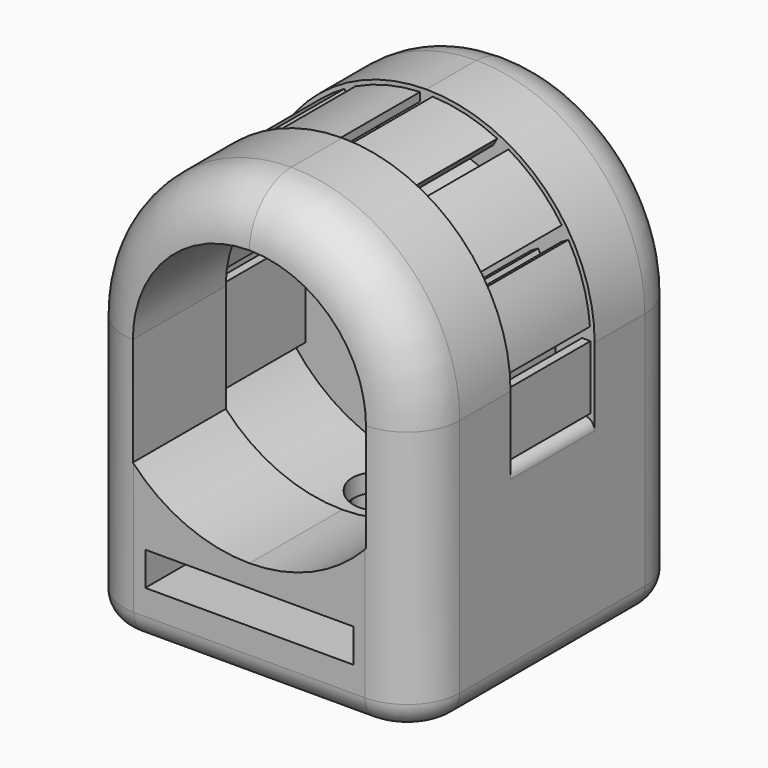
from build123d import *

# Parameters (mm, degrees)
F0_W          = 20.32
F0_H          = 20.32
F1_DEPTH      = 26.162
F2_R          = 10.15999
F3_R          = 3.2512
F4_DEPTH      = 20.321
F7_DEPTH      = 13.3604
F9_DEPTH      = 6.35
F10_R         = 0.635
F11_R         = 3.2512
F12_DEPTH     = 4.826
F13_R         = 1.905
F14_DEPTH     = 25.4
F16_W         = 12.573
F16_H         = 2.032
F17_DEPTH     = 16.51
F18_R         = 1.0795
F19_DEPTH     = 5.08
F20_T1_DEPTH  = 23.93951
F20_T3_DEPTH  = 2e-05
F20_T6_ANGLE  = 90
F20_T8_ANGLE  = 90
F20_T10_ANGLE = 90
F20_T12_ANGLE = 90
F21_R         = 1.524
F22_W         = 0.508
F22_H         = 3.8441118483
F22_H_2       = 5.6562280912
F23_DEPTH     = 6.35
F25_DEPTH     = 4.826


# Not quite as in the source:
# - a fillet or chamfer that OpenCascade refuses, or shapes differently, is made with other operations: its cross-section is extruded or revolved along the edge and cut away or added
# - a fillet or chamfer is up to 0.001 mm smaller than in the source, because OpenCascade refuses the exact size


with BuildPart() as f1:
    # F0 (on Top) → F1 (new body)
    with BuildSketch(Plane.XY):
        Rectangle(F0_W, F0_H)
    extrude(amount=F1_DEPTH)

    # F2 (radius 10.16 in the source; OpenCascade refuses exactly that, so slightly less here)
    f2_edges = [f1.edges().sort_by_distance(p)[0] for p in [
        (10.16, 0, 26.162),
        (-10.16, 0, 26.162),
    ]]
    fillet(f2_edges, radius=F2_R)

    # F3 (on face) → F4 (cut, through all)
    with BuildSketch(Plane.XZ.offset(10.16)):
        with Locations((0, 16.002)):
            Circle(F3_R)
    extrude(amount=-F4_DEPTH, mode=Mode.SUBTRACT)

    # F6 (on face) → F7 (cut)
    with BuildSketch(Plane.XZ.offset(10.16)):
        with BuildLine():
            ThreePointArc((7.0358, 16.002), (0, 23.0378), (-7.0358, 16.002))
            Line((-7.0358, 16.002), (-7.0358, 9.4689639676))
            ThreePointArc((-7.0358, 9.4689639676), (-3.8378415735, 7.2012038146), (0, 6.4008))
            ThreePointArc((0, 6.4008), (3.8378415735, 7.2012038146), (7.0358, 9.4689639676))
            Line((7.0358, 9.4689639676), (7.0358, 16.002))
        make_face()
    extrude(amount=-F7_DEPTH, mode=Mode.SUBTRACT)

    # F8 (on face) → F9 (cut)
    with BuildSketch(Plane.XZ.offset(-3.2004)):
        with BuildLine():
            Line((-12.8970071673, 11.938), (-9.1174678963, 11.938))
            ThreePointArc((-9.1174678963, 11.938), (0, 6.0198), (9.1174678963, 11.938))
            Line((9.1174678963, 11.938), (12.2319469228, 11.938))
            Line((12.2319469228, 11.938), (12.2319469228, 29.744040221))
            Line((12.2319469228, 29.744040221), (-12.8970071673, 29.744040221))
            Line((-12.8970071673, 29.744040221), (-12.8970071673, 11.938))
        make_face()
        with BuildLine():
            Line((7.0358, 16.002), (7.0358, 9.4689639676))
            ThreePointArc((7.0358, 9.4689639676), (0, 6.4008), (-7.0358, 9.4689639676))
            Line((-7.0358, 9.4689639676), (-7.0358, 16.002))
            ThreePointArc((-7.0358, 16.002), (0, 23.0378), (7.0358, 16.002))
        make_face(mode=Mode.SUBTRACT)
    extrude(amount=F9_DEPTH, mode=Mode.SUBTRACT)

    # F10
    f10_edges = [f1.edges().sort_by_distance(p)[0] for p in [
        (9.117468, 0.0254, 11.938),
        (10.16, 0.0254, 11.938),
        (-9.117468, 0.0254, 11.938),
        (-10.16, 0.0254, 11.938),
    ]]
    fillet(f10_edges, radius=F10_R)

    # F11 (on face) → F12 (cut)
    with BuildSketch(Plane(origin=(0, 10.16, 0), x_dir=(-1, 0, 0), z_dir=(0, 1, 0))):
        Polygon((-0.0026727509, 9.8428279082), (5.3326631223, 12.920099284), (5.3353358732, 19.0792713758), (0.0026727509, 22.1611720918), (-5.3326631223, 19.083900716), (-5.3353358732, 12.9247286242), align=None)
        with Locations((0, 16.002)):
            Circle(F11_R, mode=Mode.SUBTRACT)
    extrude(amount=-F12_DEPTH, mode=Mode.SUBTRACT)

    # F13 (on face) → F14 (cut)
    with BuildSketch(Plane(origin=(0, 0, 0), x_dir=(1, 0, 0), z_dir=(0, 0, -1))):
        Circle(F13_R)
    extrude(amount=-F14_DEPTH, mode=Mode.SUBTRACT)

    # F16 (on face) → F17 (cut)
    with BuildSketch(Plane.XZ.offset(10.16)):
        with Locations((0, 4.064)):
            Rectangle(F16_W, F16_H)
    extrude(amount=-F17_DEPTH, mode=Mode.SUBTRACT)

    # F18 (on face) → F19 (cut, through all)
    with BuildSketch(Plane(origin=(0, 0, 0), x_dir=(1, 0, 0), z_dir=(0, 0, -1))):
        with Locations((3.2688132281, 3.2688132281)):
            Circle(F18_R)
        with Locations((-3.2688132281, 3.2688132281)):
            Circle(F18_R)
        with Locations((-3.2688132281, -3.2688132281)):
            Circle(F18_R)
        with Locations((3.2688132281, -3.2688132281)):
            Circle(F18_R)
    extrude(amount=-F19_DEPTH, mode=Mode.SUBTRACT)

    # F20: fillet of radius 3.175 on 2 edges, made by hand

    # F20_s2 → F20_t1 (cut)
    with BuildSketch(Plane.XY.offset(-7.9375)):
        with BuildLine():
            ThreePointArc((-10.16, 6.985), (-9.2300640303, 9.2300640303), (-6.985, 10.16))
            Line((-6.985, 10.16), (-10.16, 10.16))
            Line((-10.16, 10.16), (-10.16, 6.985))
        make_face()
        with BuildLine():
            ThreePointArc((6.985, 10.16), (9.2300640303, 9.2300640303), (10.16, 6.985))
            Line((10.16, 6.985), (10.16, 10.16))
            Line((10.16, 10.16), (6.985, 10.16))
        make_face()
        with BuildLine():
            ThreePointArc((6.985, -10.16), (9.2300640303, -9.2300640303), (10.16, -6.985))
            Line((10.16, -6.985), (10.16, -10.16))
            Line((10.16, -10.16), (6.985, -10.16))
        make_face()
        with BuildLine():
            ThreePointArc((-10.16, -6.985), (-9.2300640303, -9.2300640303), (-6.985, -10.16))
            Line((-6.985, -10.16), (-10.16, -10.16))
            Line((-10.16, -10.16), (-10.16, -6.985))
        make_face()
    extrude(amount=F20_T1_DEPTH, mode=Mode.SUBTRACT)

    # F20_s4 → F20_t3 (cut)
    with BuildSketch(Plane.YZ.offset(-1e-05)):
        with BuildLine():
            ThreePointArc((10.16, 22.987), (9.2300640303, 25.2320640303), (6.985, 26.162))
            Line((6.985, 26.162), (10.16, 26.162))
            Line((10.16, 26.162), (10.16, 22.987))
        make_face()
        with BuildLine():
            ThreePointArc((-10.16, 22.987), (-9.2300640303, 25.2320640303), (-6.985, 26.162))
            Line((-6.985, 26.162), (-10.16, 26.162))
            Line((-10.16, 26.162), (-10.16, 22.987))
        make_face()
    extrude(amount=F20_T3_DEPTH, mode=Mode.SUBTRACT)

    # F20_s5 → F20_t6 (revolve, cut)
    with BuildSketch(Plane.XY.offset(16.00201)):
        with BuildLine():
            ThreePointArc((6.985, -10.16), (9.2300640303, -9.2300640303), (10.16, -6.985))
            Line((10.16, -6.985), (10.16, -10.16))
            Line((10.16, -10.16), (6.985, -10.16))
        make_face()
    revolve(axis=Axis((1e-05, -10.16, 16.00201), (0, -1, 0)), revolution_arc=F20_T6_ANGLE, mode=Mode.SUBTRACT)

    # F20_s7 → F20_t8 (revolve, cut)
    with BuildSketch(Plane.XY.offset(16.00201)):
        with BuildLine():
            ThreePointArc((-6.985, 10.16), (-9.2300640303, 9.2300640303), (-10.16, 6.985))
            Line((-10.16, 6.985), (-10.16, 10.16))
            Line((-10.16, 10.16), (-6.985, 10.16))
        make_face()
    revolve(axis=Axis((-1e-05, 10.16, 16.00201), (0, 1, 0)), revolution_arc=F20_T8_ANGLE, mode=Mode.SUBTRACT)

    # F20_s9 → F20_t10 (revolve, cut)
    with BuildSketch(Plane.XY.offset(16.00201)):
        with BuildLine():
            ThreePointArc((6.985, 10.16), (9.2300640303, 9.2300640303), (10.16, 6.985))
            Line((10.16, 6.985), (10.16, 10.16))
            Line((10.16, 10.16), (6.985, 10.16))
        make_face()
    revolve(axis=Axis((1e-05, 10.16, 16.00201), (0, -1, 0)), revolution_arc=F20_T10_ANGLE, mode=Mode.SUBTRACT)

    # F20_s11 → F20_t12 (revolve, cut)
    with BuildSketch(Plane.XY.offset(16.00201)):
        with BuildLine():
            ThreePointArc((-10.16, -6.985), (-9.2300640303, -9.2300640303), (-6.985, -10.16))
            Line((-6.985, -10.16), (-10.16, -10.16))
            Line((-10.16, -10.16), (-10.16, -6.985))
        make_face()
    revolve(axis=Axis((-1e-05, -10.16, 16.00201), (0, 1, 0)), revolution_arc=F20_T12_ANGLE, mode=Mode.SUBTRACT)

    # F21
    f21_edges = [f1.edges().sort_by_distance(p)[0] for p in [
        (10.16, 0, 0),
    ]]
    fillet(f21_edges, radius=F21_R)

    # F22 (on face) → F23 (join, through all)
    with BuildSketch(Plane(origin=(0, -3.1496, 0), x_dir=(-1, 0, 0), z_dir=(0, 1, 0))):
        with BuildLine():
            Line((9.3670571686, 16.764), (9.8766488244, 16.764))
            ThreePointArc((9.8766488244, 16.764), (9.4626876614, 18.9322522455), (8.5788476499, 20.955))
            Line((8.5788476499, 20.955), (8.1389067448, 20.701))
            ThreePointArc((8.1389067448, 20.701), (8.971604393, 18.8006994508), (9.3670571686, 16.764))
        make_face()
        with Locations((-9.652, 14.0799440759)):
            Rectangle(F22_W, F22_H)
        with Locations((9.652, 14.0799440759)):
            Rectangle(F22_W, F22_H)
        with Locations((7.5438, 13.1738859544)):
            Rectangle(F22_W, F22_H_2)
        with BuildLine():
            Line((-7.7604794208, 16.764), (-7.2498648291, 16.764))
            ThreePointArc((-7.2498648291, 16.764), (-6.9330104862, 18.2546761061), (-6.3131519885, 19.6469))
            Line((-6.3131519885, 19.6469), (-6.7530928936, 19.9009))
            ThreePointArc((-6.7530928936, 19.9009), (-7.4243505261, 18.3862617529), (-7.7604794208, 16.764))
        make_face()
        Polygon((-7.2898, 10.0334273864), (-7.2898, 16.002), (-7.7978, 16.002), (-7.7978, 10.022544302), align=None)
        with BuildLine():
            ThreePointArc((6.3131519885, 19.6469), (6.9330104862, 18.2546761061), (7.2498648291, 16.764))
            Line((7.2498648291, 16.764), (7.7604794208, 16.764))
            ThreePointArc((7.7604794208, 16.764), (7.4243505261, 18.3862617529), (6.7530928936, 19.9009))
            Line((6.7530928936, 19.9009), (6.3131519885, 19.6469))
        make_face()
        with BuildLine():
            Line((-9.8766488244, 16.764), (-9.3670571686, 16.764))
            ThreePointArc((-9.3670571686, 16.764), (-8.971604393, 18.8006994508), (-8.1389067448, 20.701))
            Line((-8.1389067448, 20.701), (-8.5788476499, 20.955))
            ThreePointArc((-8.5788476499, 20.955), (-9.4626876614, 18.9322522455), (-9.8766488244, 16.764))
        make_face()
        with BuildLine():
            Line((0.381, 23.7904866206), (0.381, 23.2818367454))
            ThreePointArc((0.381, 23.2818367454), (1.7015133945, 23.0904438496), (2.9650210569, 22.661567116))
            Line((2.9650210569, 22.661567116), (3.2203283527, 23.1037723239))
            ThreePointArc((3.2203283527, 23.1037723239), (1.8331081821, 23.581274321), (0.381, 23.7904866206))
        make_face()
        with BuildLine():
            ThreePointArc((-2.9650210569, 22.661567116), (-1.7015133945, 23.0904438496), (-0.381, 23.2818367454))
            Line((-0.381, 23.2818367454), (-0.381, 23.7904866206))
            ThreePointArc((-0.381, 23.7904866206), (-1.8331081821, 23.581274321), (-3.2203283527, 23.1037723239))
            Line((-3.2203283527, 23.1037723239), (-2.9650210569, 22.661567116))
        make_face()
        with BuildLine():
            ThreePointArc((-4.0236172266, 24.4951094667), (-2.2475295797, 25.1272953261), (-0.381, 25.3922738512))
            Line((-0.381, 25.3922738512), (-0.381, 25.9006703653))
            ThreePointArc((-0.381, 25.9006703653), (-2.3790697675, 25.6180731612), (-4.2784130545, 24.9364287862))
            Line((-4.2784130545, 24.9364287862), (-4.0236172266, 24.4951094667))
        make_face()
        with BuildLine():
            Line((0.381, 25.9006703653), (0.381, 25.3922738512))
            ThreePointArc((0.381, 25.3922738512), (2.2475295797, 25.1272953261), (4.0236172266, 24.4951094667))
            Line((4.0236172266, 24.4951094667), (4.2784130545, 24.9364287862))
            ThreePointArc((4.2784130545, 24.9364287862), (2.3790697675, 25.6180731612), (0.381, 25.9006703653))
        make_face()
        with BuildLine():
            ThreePointArc((4.699, 24.1409067448), (6.3702875916, 22.9115470184), (7.7311094667, 21.345439942))
            Line((7.7311094667, 21.345439942), (8.1724287862, 21.6002357699))
            ThreePointArc((8.1724287862, 21.6002357699), (6.7298017801, 23.2710167148), (4.953, 24.5808476499))
            Line((4.953, 24.5808476499), (4.699, 24.1409067448))
        make_face()
        with BuildLine():
            ThreePointArc((3.6449, 22.3151519885), (4.8778251527, 21.4193799774), (5.897567116, 20.2868437722))
            Line((5.897567116, 20.2868437722), (6.3397723239, 20.5421510681))
            ThreePointArc((6.3397723239, 20.5421510681), (5.2375452857, 21.7790065103), (3.8989, 22.7550928936))
            Line((3.8989, 22.7550928936), (3.6449, 22.3151519885))
        make_face()
        with BuildLine():
            ThreePointArc((-5.897567116, 20.2868437722), (-4.8778251527, 21.4193799774), (-3.6449, 22.3151519885))
            Line((-3.6449, 22.3151519885), (-3.8989, 22.7550928936))
            ThreePointArc((-3.8989, 22.7550928936), (-5.2375452857, 21.7790065103), (-6.3397723239, 20.5421510681))
            Line((-6.3397723239, 20.5421510681), (-5.897567116, 20.2868437722))
        make_face()
        with BuildLine():
            ThreePointArc((-7.7311094667, 21.345439942), (-6.3702875916, 22.9115470184), (-4.699, 24.1409067448))
            Line((-4.699, 24.1409067448), (-4.953, 24.5808476499))
            ThreePointArc((-4.953, 24.5808476499), (-6.7298017801, 23.2710167148), (-8.1724287862, 21.6002357699))
            Line((-8.1724287862, 21.6002357699), (-7.7311094667, 21.345439942))
        make_face()
    extrude(amount=F23_DEPTH)

    # F24 (on face) → F25 (join, through all)
    with BuildSketch(Plane(origin=(0, 5.334, 0), x_dir=(-1, 0, 0), z_dir=(0, 1, 0))):
        Polygon((-0.6368127329, 21.0592836333), (-4.4437586614, 18.8635445058), (-4.1899495961, 18.4234934198), (-0.3830036675, 20.6192325472), align=None)
        Polygon((4.6982802155, 14.3422860637), (4.6997206697, 17.6617145614), (4.1917205262, 17.6614941165), (4.1902802633, 14.3425065085), align=None)
        Polygon((4.4427103254, 18.8617269135), (0.6331854257, 21.0633618652), (0.3789945388, 20.6235312239), (4.1920496147, 18.4198560809), align=None)
        Polygon((-4.6982802155, 17.6617139363), (-4.6997206697, 14.3422854386), (-4.1917205262, 14.3425058835), (-4.1902802633, 17.6614934915), align=None)
        Polygon((-0.3830036675, 11.3847674528), (-4.1899495961, 13.5805065802), (-4.4437586614, 13.1404554942), (-0.6368127329, 10.9447163667), align=None)
        Polygon((4.4427103254, 13.1422730865), (4.1920496147, 13.5841439191), (0.3789945388, 11.3804687761), (0.6331854257, 10.9406381348), align=None)
    extrude(amount=F25_DEPTH)


solid = f1.part
